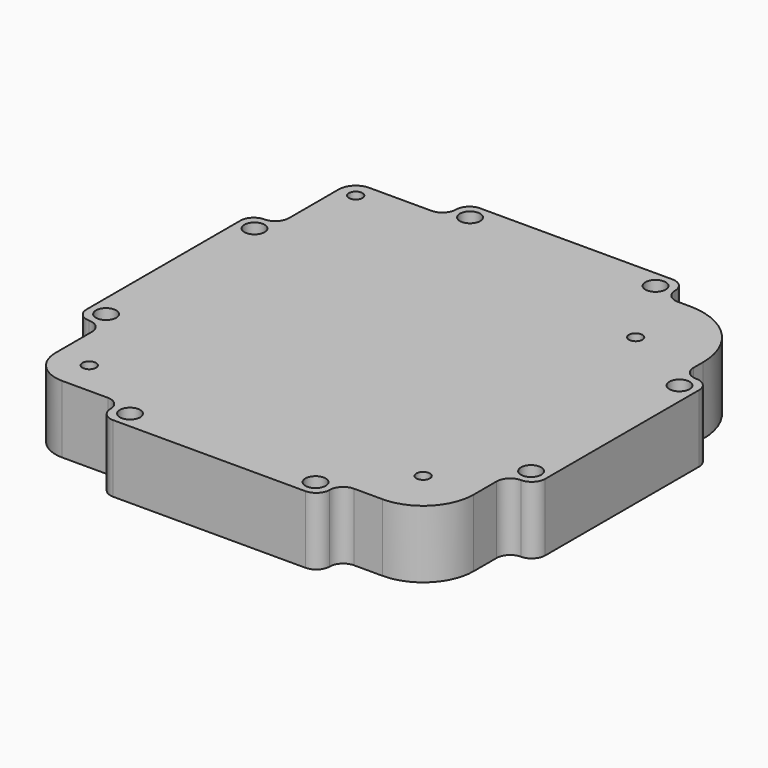
from build123d import *

# Parameters (mm, degrees)
F0_R     = 2
F0_R_2   = 3
F1_DEPTH = 20
F2_R     = 3.99999


# Not quite as in the source:
# - a fillet or chamfer is up to 0.001 mm smaller than in the source, because OpenCascade refuses the exact size


with BuildPart() as f1:
    # F0 (on Top) → F1 (new body)
    with BuildSketch(Plane.XY):
        with BuildLine():
            Line((-32.5, 60), (-55, 60))
            ThreePointArc((-55, 60), (-58.5355339059, 58.5355339059), (-60, 55))
            Line((-60, 55), (-60, 32.5))
            Line((-60, 32.5), (-68, 32.5))
            Line((-68, 32.5), (-68, -32.5))
            Line((-68, -32.5), (-60, -32.5))
            Line((-60, -32.5), (-60, -50))
            ThreePointArc((-60, -50), (-57.0710678119, -57.0710678119), (-50, -60))
            Line((-50, -60), (-32.5, -60))
            Line((-32.5, -60), (-32.5, -68))
            Line((-32.5, -68), (32.5, -68))
            Line((32.5, -68), (32.5, -60))
            Line((32.5, -60), (45, -60))
            ThreePointArc((45, -60), (55.6066017178, -55.6066017178), (60, -45))
            Line((60, -45), (60, -32.5))
            Line((60, -32.5), (68, -32.5))
            Line((68, -32.5), (68, 32.5))
            Line((68, 32.5), (60, 32.5))
            Line((60, 32.5), (60, 40))
            ThreePointArc((60, 40), (54.1421356237, 54.1421356237), (40, 60))
            Line((40, 60), (32.5, 60))
            Line((32.5, 60), (32.5, 68))
            Line((32.5, 68), (-32.5, 68))
            Line((-32.5, 68), (-32.5, 60))
        make_face()
        with Locations((-50, -50)):
            Circle(F0_R, mode=Mode.SUBTRACT)
        with Locations((-27.5, -63)):
            Circle(F0_R_2, mode=Mode.SUBTRACT)
        with Locations((-63, -27.5)):
            Circle(F0_R_2, mode=Mode.SUBTRACT)
        with Locations((27.5, -63)):
            Circle(F0_R_2, mode=Mode.SUBTRACT)
        with Locations((45, -45)):
            Circle(F0_R, mode=Mode.SUBTRACT)
        with Locations((63, -27.5)):
            Circle(F0_R_2, mode=Mode.SUBTRACT)
        with Locations((-63, 27.5)):
            Circle(F0_R_2, mode=Mode.SUBTRACT)
        with Locations((-55, 55)):
            Circle(F0_R, mode=Mode.SUBTRACT)
        with Locations((-27.5, 63)):
            Circle(F0_R_2, mode=Mode.SUBTRACT)
        with Locations((63, 27.5)):
            Circle(F0_R_2, mode=Mode.SUBTRACT)
        with Locations((27.5, 63)):
            Circle(F0_R_2, mode=Mode.SUBTRACT)
        with Locations((40, 40)):
            Circle(F0_R, mode=Mode.SUBTRACT)
    extrude(amount=F1_DEPTH)

    # F2 (radius 4 in the source; OpenCascade refuses exactly that, so slightly less here)
    f2_edges = [f1.edges().sort_by_distance(p)[0] for p in [
        (-60, 32.5, 10),
        (-68, 32.5, 10),
        (-32.5, 60, 10),
        (-32.5, 68, 10),
        (32.5, 68, 10),
        (-68, -32.5, 10),
        (-32.5, -68, 10),
        (60, -32.5, 10),
        (68, -32.5, 10),
        (68, 32.5, 10),
        (32.5, -60, 10),
        (32.5, -68, 10),
        (-60, -32.5, 10),
        (-32.5, -60, 10),
        (60, 32.5, 10),
        (32.5, 60, 10),
    ]]
    fillet(f2_edges, radius=F2_R)


solid = f1.part
